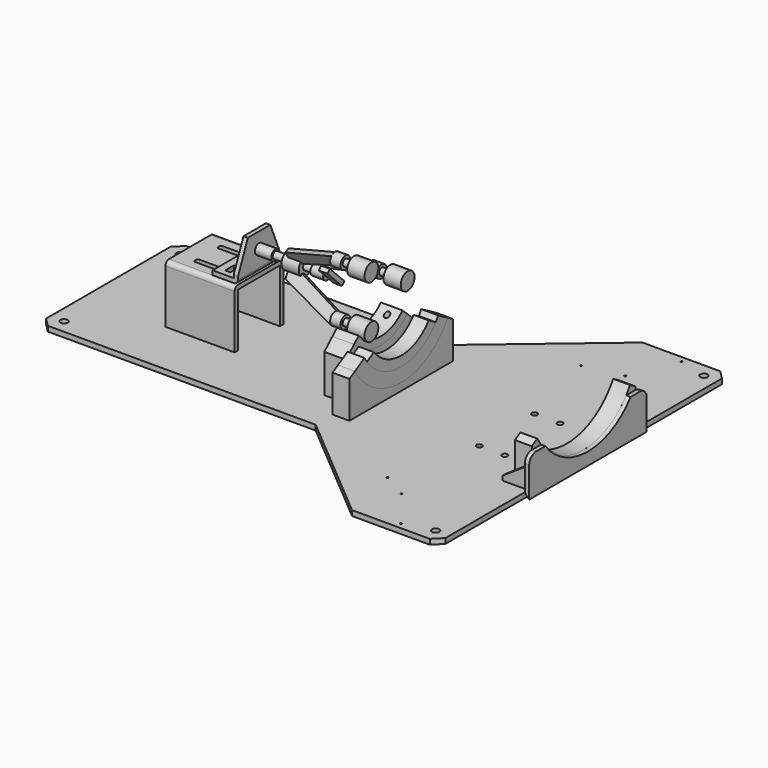
from build123d import *

# Parameters (mm, degrees)
F0_R      = 1
F0_R_2    = 3.2
F1_DEPTH  = 6
F3_W      = 29.5
F3_H      = 60.5
F3_W_2    = 6
F3_H_2    = 13
F4_DEPTH  = 5
F6_DEPTH  = 5
F7_R      = 5
F8_R      = 6
F8_R_2    = 4
F9_DEPTH  = 19
F10_R     = 4
F11_DEPTH = 15
F12_DEPTH = 15
F13_R     = 10
F13_R_2   = 4
F14_DEPTH = 20
F15_R     = 4
F16_DEPTH = 15
F17_DEPTH = 15
F18_R     = 4
F19_DEPTH = 10
F20_DEPTH = 20
F22_R     = 6
F23_DEPTH = 15
F25_DEPTH = 10
F26_ANGLE = 45
F28_R     = 10
F29_DEPTH = 20
F30_R     = 4
F31_DEPTH = 20
F33_R     = 7.2
F33_R_2   = 4
F34_DEPTH = 12
F35_W     = 15
F35_H     = 2.6824583655
F36_DEPTH = 5
F37_ANGLE = 120
F38_ANGLE = -120
F40_DEPTH = 19.5
F41_W     = 6
F41_H     = 3.5
F41_W_2   = 5
F41_H_2   = 60.5
F42_DEPTH = 5
F43_W     = 80
F43_H     = 62
F44_DEPTH = 5
F45_R     = 4.99999
F46_W     = 80
F46_H     = 62
F47_DEPTH = 5
F48_R     = 4.99999
F50_DEPTH = 5
F51_SIZE  = 4.99999
F53_DEPTH = 5
F57_DEPTH = 19.5
F58_DEPTH = 17.5
F61_DEPTH = 25
F62_DEPTH = 25
F63_DEPTH = 25
F64_R     = 3
F65_DEPTH = 137.3118891325
F64_R_2   = 4.25
F66_DEPTH = 25


# Not quite as in the source:
# - a fillet or chamfer is up to 0.001 mm smaller than in the source, because OpenCascade refuses the exact size


with BuildPart() as f1:
    # F0 (on Top) → F1 (new body)
    with BuildSketch(Plane.XY):
        Polygon((230, -200), (230, 200), (220, 210), (130, 210), (0, 100), (-310, 100), (-320, 90), (-320, -90), (-310, -100), (0, -100), (130, -210), (220, -210), align=None)
        with Locations((181, -203)):
            Circle(F0_R, mode=Mode.SUBTRACT)
        with Locations((115, -140)):
            Circle(F0_R, mode=Mode.SUBTRACT)
        with Locations((145, -157)):
            Circle(F0_R, mode=Mode.SUBTRACT)
        with Locations((8.75, -40)):
            Circle(F0_R_2, mode=Mode.SUBTRACT)
        with Locations((141.25, -40)):
            Circle(F0_R_2, mode=Mode.SUBTRACT)
        with Locations((170.75, -40)):
            Circle(F0_R_2, mode=Mode.SUBTRACT)
        with Locations((219.75, -40)):
            Circle(F0_R_2, mode=Mode.SUBTRACT)
        with Locations((8.75, 40)):
            Circle(F0_R_2, mode=Mode.SUBTRACT)
        with Locations((141.25, 40)):
            Circle(F0_R_2, mode=Mode.SUBTRACT)
        with Locations((170.75, 40)):
            Circle(F0_R_2, mode=Mode.SUBTRACT)
        with Locations((219.75, 40)):
            Circle(F0_R_2, mode=Mode.SUBTRACT)
        with Locations((115, 140)):
            Circle(F0_R, mode=Mode.SUBTRACT)
        with Locations((158.6559563875, 149.430975318)):
            Circle(F0_R, mode=Mode.SUBTRACT)
        with Locations((181, 203)):
            Circle(F0_R, mode=Mode.SUBTRACT)
    extrude(amount=F1_DEPTH)



with BuildPart() as f4:
    # F3 (on offset) → F4 (new body)
    with BuildSketch(Plane.XY.offset(73)):
        with Locations((-160.3453308344, 0)):
            Rectangle(F3_W, F3_H)
        with Locations((-163.0953308344, -16.8823601156)):
            Rectangle(F3_W_2, F3_H_2, mode=Mode.SUBTRACT)
        with Locations((-162.4798774719, 16.8823601156)):
            Rectangle(F3_W_2, F3_H_2, mode=Mode.SUBTRACT)
    extrude(amount=F4_DEPTH)

    # F5 (on face) → F6 (join)
    with BuildSketch(Plane.YZ.offset(-145.5953308344)):
        Polygon((-30.25, 78), (30.25, 78), (30.25, 81.6910490394), (16.2317510694, 115), (-16.2317510694, 115), (-30.25, 81.6910490394), align=None)
    extrude(amount=-F6_DEPTH)

    # F7
    f7_edges = [f4.edges().sort_by_distance(p)[0] for p in [
        (-145.595331, 0, 73),
    ]]
    fillet(f7_edges, radius=F7_R)

    # F41 (on face) → F42 (join)
    with BuildSketch(Plane(origin=(0, 0, 73), x_dir=(1, 0, 0), z_dir=(0, 0, -1))):
        with BuildLine():
            Line((-175.0953308344, 19.8823601156), (-175.0953308344, 30.25))
            Line((-175.0953308344, 30.25), (-225.5953308344, 30.25))
            Line((-225.5953308344, 30.25), (-225.5953308344, -30.25))
            Line((-225.5953308344, -30.25), (-175.0953308344, -30.25))
            Line((-175.0953308344, -30.25), (-175.0953308344, -19.8823601156))
            Line((-175.0953308344, -19.8823601156), (-203.5953308344, -19.8823601156))
            ThreePointArc((-203.5953308344, -19.8823601156), (-205.0095443968, -19.296573678), (-205.5953308344, -17.8823601156))
            Line((-205.5953308344, -17.8823601156), (-205.5953308344, -15.8823601156))
            ThreePointArc((-205.5953308344, -15.8823601156), (-205.0095443968, -14.4681465533), (-203.5953308344, -13.8823601156))
            Line((-203.5953308344, -13.8823601156), (-175.0953308344, -13.8823601156))
            Line((-175.0953308344, -13.8823601156), (-175.0953308344, 13.8823601156))
            Line((-175.0953308344, 13.8823601156), (-203.5953308344, 13.8823601156))
            ThreePointArc((-203.5953308344, 13.8823601156), (-205.0095443968, 14.4681465533), (-205.5953308344, 15.8823601156))
            Line((-205.5953308344, 15.8823601156), (-205.5953308344, 17.8823601156))
            ThreePointArc((-205.5953308344, 17.8823601156), (-205.0095443968, 19.296573678), (-203.5953308344, 19.8823601156))
            Line((-203.5953308344, 19.8823601156), (-175.0953308344, 19.8823601156))
        make_face()
        with BuildLine():
            Line((-150.5953308344, -30.25), (-150.5953308344, 30.25))
            Line((-150.5953308344, 30.25), (-175.0953308344, 30.25))
            Line((-175.0953308344, 30.25), (-175.0953308344, 19.8823601156))
            Line((-175.0953308344, 19.8823601156), (-166.0953308344, 19.8823601156))
            Line((-166.0953308344, 19.8823601156), (-166.0953308344, 23.3823601156))
            Line((-166.0953308344, 23.3823601156), (-160.0953308344, 23.3823601156))
            Line((-160.0953308344, 23.3823601156), (-160.0953308344, 19.8823601156))
            Line((-160.0953308344, 19.8823601156), (-157.5953308344, 19.8823601156))
            ThreePointArc((-157.5953308344, 19.8823601156), (-156.181117272, 19.296573678), (-155.5953308344, 17.8823601156))
            Line((-155.5953308344, 17.8823601156), (-155.5953308344, 15.8823601156))
            ThreePointArc((-155.5953308344, 15.8823601156), (-156.181117272, 14.4681465533), (-157.5953308344, 13.8823601156))
            Line((-157.5953308344, 13.8823601156), (-160.0953308344, 13.8823601156))
            Line((-160.0953308344, 13.8823601156), (-160.0953308344, 10.3823601156))
            Line((-160.0953308344, 10.3823601156), (-166.0953308344, 10.3823601156))
            Line((-166.0953308344, 10.3823601156), (-166.0953308344, 13.8823601156))
            Line((-166.0953308344, 13.8823601156), (-175.0953308344, 13.8823601156))
            Line((-175.0953308344, 13.8823601156), (-175.0953308344, -13.8823601156))
            Line((-175.0953308344, -13.8823601156), (-165.4798774719, -13.8823601156))
            Line((-165.4798774719, -13.8823601156), (-165.4798774719, -10.3823601156))
            Line((-165.4798774719, -10.3823601156), (-159.4798774719, -10.3823601156))
            Line((-159.4798774719, -10.3823601156), (-159.4798774719, -13.8823601156))
            Line((-159.4798774719, -13.8823601156), (-157.5953308344, -13.8823601156))
            ThreePointArc((-157.5953308344, -13.8823601156), (-156.181117272, -14.4681465533), (-155.5953308344, -15.8823601156))
            Line((-155.5953308344, -15.8823601156), (-155.5953308344, -17.8823601156))
            ThreePointArc((-155.5953308344, -17.8823601156), (-156.181117272, -19.296573678), (-157.5953308344, -19.8823601156))
            Line((-157.5953308344, -19.8823601156), (-159.4798774719, -19.8823601156))
            Line((-159.4798774719, -19.8823601156), (-159.4798774719, -23.3823601156))
            Line((-159.4798774719, -23.3823601156), (-165.4798774719, -23.3823601156))
            Line((-165.4798774719, -23.3823601156), (-165.4798774719, -19.8823601156))
            Line((-165.4798774719, -19.8823601156), (-175.0953308344, -19.8823601156))
            Line((-175.0953308344, -19.8823601156), (-175.0953308344, -30.25))
            Line((-175.0953308344, -30.25), (-150.5953308344, -30.25))
        make_face()
        with Locations((-162.4798774719, -21.6323601156)):
            Rectangle(F41_W, F41_H)
        with Locations((-162.4798774719, -12.1323601156)):
            Rectangle(F41_W, F41_H)
        with Locations((-163.0953308344, 12.1323601156)):
            Rectangle(F41_W, F41_H)
        with Locations((-163.0953308344, 21.6323601156)):
            Rectangle(F41_W, F41_H)
        with Locations((-148.0953308344, 0)):
            Rectangle(F41_W_2, F41_H_2)
    extrude(amount=F42_DEPTH)


with BuildPart() as f9:
    # F8 (on face) → F9 (new body)
    with BuildSketch(Plane.YZ.offset(-145.5953308344)):
        with Locations((0, 97)):
            Circle(F8_R)
        with Locations((0, 97)):
            Circle(F8_R_2, mode=Mode.SUBTRACT)
    extrude(amount=F9_DEPTH)


with BuildPart() as f11:
    # F10 (on face) → F11 (new body)
    with BuildSketch(Plane.YZ.offset(-126.5953308344)):
        with Locations((0, 97)):
            Circle(F10_R)
    extrude(amount=-F11_DEPTH)

    # F12 (add): a face of the model
    f12_faces = [f11.faces().sort_by_distance(p)[0] for p in [
        (-126.5953308344, 0, 97),
    ]]
    extrude(f12_faces, amount=F12_DEPTH)

    # F13 (on face) → F14 (join)
    with BuildSketch(Plane.YZ.offset(-111.5953308344)):
        with Locations((0, 97)):
            Circle(F13_R)
        with Locations((0, 97)):
            Circle(F13_R_2, mode=Mode.SUBTRACT)
        with Locations((0, 97)):
            Circle(F13_R_2)
    extrude(amount=F14_DEPTH)

    # F15 (on face) → F16 (cut)
    with BuildSketch(Plane.YZ.offset(-91.5953308344)):
        with Locations((0, 97)):
            Circle(F15_R)
    extrude(amount=-F16_DEPTH, mode=Mode.SUBTRACT)

    # F15 (on face) → F17 (cut)
    with BuildSketch(Plane.YZ.offset(-91.5953308344)):
        with BuildLine():
            ThreePointArc((-2.6761656733, 106.6352549156), (-5, 105.6602540378), (-7.0062926922, 104.1352549156))
            Line((-7.0062926922, 104.1352549156), (-5.6650635095, 101.8121778265))
            Line((-5.6650635095, 101.8121778265), (-1.3349364905, 104.3121778265))
            Line((-1.3349364905, 104.3121778265), (-2.6761656733, 106.6352549156))
        make_face()
        with BuildLine():
            ThreePointArc((-7.0062926922, 89.8647450844), (-5, 88.3397459622), (-2.6761656733, 87.3647450844))
            Line((-2.6761656733, 87.3647450844), (-1.3349364905, 89.6878221735))
            Line((-1.3349364905, 89.6878221735), (-5.6650635095, 92.1878221735))
            Line((-5.6650635095, 92.1878221735), (-7.0062926922, 89.8647450844))
        make_face()
        with BuildLine():
            Line((7, 94.5), (9.6824583655, 94.5))
            ThreePointArc((9.6824583655, 94.5), (9.9202969627, 95.7399570752), (10, 97))
            ThreePointArc((10, 97), (9.9202969627, 98.2600429248), (9.6824583655, 99.5))
            Line((9.6824583655, 99.5), (7, 99.5))
            Line((7, 99.5), (7, 94.5))
        make_face()
    extrude(amount=-F17_DEPTH, mode=Mode.SUBTRACT)


with BuildPart() as f19:
    # F18 (on face) → F19 (new body)
    with BuildSketch(Plane.YZ.offset(-91.5953308344)):
        with Locations((0, 97)):
            Circle(F18_R)
    extrude(amount=-F19_DEPTH)

    # F20 (add): a face of the model
    f20_faces = [f19.faces().sort_by_distance(p)[0] for p in [
        (-91.5953308344, 0, 97),
    ]]
    extrude(f20_faces, amount=F20_DEPTH)


with BuildPart() as f23:
    # F22 (on offset) → F23 (new body)
    with BuildSketch(Plane.YZ.offset(-81.5953308344)):
        with Locations((0, 97)):
            Circle(F22_R)
    extrude(amount=F23_DEPTH)

    # F24 (on face) → F25 (join)
    with BuildSketch(Plane.YZ.offset(-66.5953308344)):
        with BuildLine():
            Line((2.5, 112), (-2.5, 112))
            Line((-2.5, 112), (-2.5, 102.4543560573))
            ThreePointArc((-2.5, 102.4543560573), (0, 103), (2.5, 102.4543560573))
            Line((2.5, 102.4543560573), (2.5, 112))
        make_face()
        with BuildLine():
            ThreePointArc((2.5, 102.4543560573), (0, 103), (-2.5, 102.4543560573))
            Line((-2.5, 102.4543560573), (-2.5, 91.5456439427))
            ThreePointArc((-2.5, 91.5456439427), (0, 91), (2.5, 91.5456439427))
            Line((2.5, 91.5456439427), (2.5, 102.4543560573))
        make_face()
        with BuildLine():
            ThreePointArc((2.5, 91.5456439427), (0, 91), (-2.5, 91.5456439427))
            Line((-2.5, 91.5456439427), (-2.5, 82))
            Line((-2.5, 82), (2.5, 82))
            Line((2.5, 82), (2.5, 91.5456439427))
        make_face()
    extrude(amount=F25_DEPTH)


with BuildPart() as f23_1:
    # F26: moved
    add(f23.part.rotate(Axis((-91.5953308344, 0, 97), (1, 0, 0)), F26_ANGLE))


with BuildPart() as f29:
    # F28 (on offset) → F29 (new body)
    with BuildSketch(Plane.YZ.offset(-1.5953308344)):
        with Locations((-17.5, 127.3108891325)):
            Circle(F28_R)
    extrude(amount=-F29_DEPTH)


with BuildPart() as f29b:
    # F28 (on offset) → F29, piece 2 (new body)
    with BuildSketch(Plane.YZ.offset(-1.5953308344)):
        with Locations((35, 97)):
            Circle(F28_R)
    extrude(amount=-F29_DEPTH)


with BuildPart() as f29c:
    # F28 (on offset) → F29, piece 3 (new body)
    with BuildSketch(Plane.YZ.offset(-1.5953308344)):
        with Locations((-17.5, 66.6891108675)):
            Circle(F28_R)
    extrude(amount=-F29_DEPTH)


with BuildPart() as f31:
    # F30 (on face) → F31 (new body)
    with BuildSketch(Plane(origin=(-21.5953308344, 0, 0), x_dir=(0, -1, 0), z_dir=(-1, 0, 0))):
        with Locations((17.5, 66.6891108675)):
            Circle(F30_R)
    extrude(amount=F31_DEPTH)


with BuildPart() as f31b:
    # F30 (on face) → F31, piece 2 (new body)
    with BuildSketch(Plane(origin=(-21.5953308344, 0, 0), x_dir=(0, -1, 0), z_dir=(-1, 0, 0))):
        with Locations((-35, 97)):
            Circle(F30_R)
    extrude(amount=F31_DEPTH)


with BuildPart() as f31c:
    # F30 (on face) → F31, piece 3 (new body)
    with BuildSketch(Plane(origin=(-21.5953308344, 0, 0), x_dir=(0, -1, 0), z_dir=(-1, 0, 0))):
        with Locations((17.5, 127.3108891325)):
            Circle(F30_R)
    extrude(amount=F31_DEPTH)


with BuildPart() as f34:
    # F33 (on offset) → F34 (new body)
    with BuildSketch(Plane(origin=(-31.5953308344, 0, 0), x_dir=(0, -1, 0), z_dir=(-1, 0, 0))):
        with Locations((17.5, 127.3108891325)):
            Circle(F33_R)
        with Locations((17.5, 127.3108891325)):
            Circle(F33_R_2, mode=Mode.SUBTRACT)
    extrude(amount=F34_DEPTH)


with BuildPart() as f34b:
    # F33 (on offset) → F34, piece 2 (new body)
    with BuildSketch(Plane(origin=(-31.5953308344, 0, 0), x_dir=(0, -1, 0), z_dir=(-1, 0, 0))):
        with Locations((17.5, 66.6891108675)):
            Circle(F33_R)
        with Locations((17.5, 66.6891108675)):
            Circle(F33_R_2, mode=Mode.SUBTRACT)
    extrude(amount=F34_DEPTH)


with BuildPart() as f34c:
    # F33 (on offset) → F34, piece 3 (new body)
    with BuildSketch(Plane(origin=(-31.5953308344, 0, 0), x_dir=(0, -1, 0), z_dir=(-1, 0, 0))):
        with Locations((-35, 97)):
            Circle(F33_R)
        with Locations((-35, 97)):
            Circle(F33_R_2, mode=Mode.SUBTRACT)
    extrude(amount=F34_DEPTH)


with BuildPart() as f36:
    # F35 (on face) → F36 (new body)
    with BuildSketch(Plane(origin=(0, 39.8371685741, 23), x_dir=(-1, 0, 0), z_dir=(0, 0.8660254038, 0.5))):
        Polygon((43.5953308344, 111.8044641671), (91.5953308344, 91.0044641671), (91.5953308344, 93.6869225326), (106.5953308344, 93.6869225326), (106.5953308344, 101.0044641671), (43.5953308344, 126.2044641671), align=None)
        with Locations((99.0953308344, 92.3456933498)):
            Rectangle(F35_W, F35_H)
    extrude(amount=F36_DEPTH)


with BuildPart() as f37_1:
    # F37: copy of F36
    add(f36.part.rotate(Axis((-111.5953308344, 0, 97), (-1, 0, 0)), F37_ANGLE))


with BuildPart() as f38_1:
    # F38: copy of F36
    add(f36.part.rotate(Axis((-111.5953308344, 0, 97), (-1, 0, 0)), F38_ANGLE))


with BuildPart() as f40:
    # F39 (on face) → F40 (new body)
    with BuildSketch(Plane.YZ.offset(230)):
        with BuildLine():
            Line((-75, 48.6987298108), (-75, 6))
            Line((-75, 6), (75, 6))
            Line((75, 6), (75, 48.6987298108))
            Line((75, 48.6987298108), (67.1169687933, 53.25))
            ThreePointArc((67.1169687933, 53.25), (0, 14.5), (-67.1169687933, 53.25))
            Line((-67.1169687933, 53.25), (-75, 48.6987298108))
        make_face()
    extrude(amount=-F40_DEPTH)


with BuildPart() as f1_1:
    add(f1.part)

    add(f4.part)  # F44 merges F4
    # F43 (on face) → F44 (join)
    with BuildSketch(Plane.XZ.offset(30.25)):
        with Locations((-185.5953308344, 37)):
            Rectangle(F43_W, F43_H)
        Polygon((-145.5953308344, 68), (-145.5953308344, 73), (-150.5953308344, 73), (-175.0953308344, 73), (-225.5953308344, 73), (-225.5953308344, 68), align=None)
    extrude(amount=F44_DEPTH)

    # F45 (radius 5 in the source; OpenCascade refuses exactly that, so slightly less here)
    f45_edges = [f1_1.edges().sort_by_distance(p)[0] for p in [
        (-185.595331, -35.25, 73),
    ]]
    fillet(f45_edges, radius=F45_R)

    # F46 (on face) → F47 (join)
    with BuildSketch(Plane(origin=(0, 30.25, 0), x_dir=(-1, 0, 0), z_dir=(0, 1, 0))):
        with Locations((185.5953308344, 37)):
            Rectangle(F46_W, F46_H)
        Polygon((225.5953308344, 68), (225.5953308344, 73), (175.0953308344, 73), (150.5953308344, 73), (145.5953308344, 73), (145.5953308344, 68), align=None)
    extrude(amount=F47_DEPTH)

    # F48 (radius 5 in the source; OpenCascade refuses exactly that, so slightly less here)
    f48_edges = [f1_1.edges().sort_by_distance(p)[0] for p in [
        (-185.595331, 35.25, 73),
    ]]
    fillet(f48_edges, radius=F48_R)


with BuildPart() as f50:
    # F49 (on face) → F50 (new body)
    with BuildSketch(Plane.YZ.offset(230)):
        with BuildLine():
            Line((-85, 0), (85, 0))
            Line((85, 0), (85, 35))
            ThreePointArc((85, 35), (82.0710678119, 42.0710678119), (75, 45))
            Line((75, 45), (75, 6))
            Line((75, 6), (-75, 6))
            Line((-75, 6), (-75, 45))
            ThreePointArc((-75, 45), (-82.0710678119, 42.0710678119), (-85, 35))
            Line((-85, 35), (-85, 0))
        make_face()
        with BuildLine():
            Line((75, 6), (75, 45))
            Line((75, 45), (61.6218305473, 45))
            ThreePointArc((61.6218305473, 45), (0, 14.5), (-61.6218305473, 45))
            Line((-61.6218305473, 45), (-75, 45))
            Line((-75, 45), (-75, 6))
            Line((-75, 6), (75, 6))
        make_face()
    extrude(amount=F50_DEPTH)

    # F51 (size 5 in the source; OpenCascade refuses exactly that, so slightly less here)
    f51_edges = [f50.edges().sort_by_distance(p)[0] for p in [
        (230, 0, 0),
    ]]
    chamfer(f51_edges, length=F51_SIZE)


with BuildPart() as f53:
    # F52 (on face) → F53 (new body)
    with BuildSketch(Plane.XZ.offset(75)):
        Polygon((200, 6), (210.5, 6), (210.5, 18), (200, 11), align=None)
        Polygon((210.5, 6), (230, 6), (230, 31), (210.5, 18), align=None)
    extrude(amount=F53_DEPTH)


with BuildPart() as f54_1:
    # F54: copy of F53
    add(f53.part.moved(Location((0, 155, 0))))


with BuildPart() as f55_1:
    # F55: copy of F40
    add(f40.part.moved(Location((-211, 0, 0))))


with BuildPart() as f57:
    # F56 (on face) → F57 (new body)
    with BuildSketch(Plane.YZ.offset(19)):
        with BuildLine():
            Line((-53.2605623327, 61.25), (-67.1169687933, 53.25))
            ThreePointArc((-67.1169687933, 53.25), (0, 14.5), (67.1169687933, 53.25))
            Line((67.1169687933, 53.25), (53.2605623327, 61.25))
            ThreePointArc((53.2605623327, 61.25), (51.5597557341, 58.4762533621), (49.7146348004, 55.7963387671))
            ThreePointArc((49.7146348004, 55.7963387671), (0, 30.5), (-49.7146348004, 55.7963387671))
            ThreePointArc((-49.7146348004, 55.7963387671), (-51.5597557341, 58.4762533621), (-53.2605623327, 61.25))
        make_face()
    extrude(amount=-F57_DEPTH)


with BuildPart() as f58:
    # F56 (on face) → F58 (new body)
    with BuildSketch(Plane.YZ.offset(19)):
        with BuildLine():
            Line((-39.6862859915, 61.5862086514), (-49.7146348004, 55.7963387671))
            ThreePointArc((-49.7146348004, 55.7963387671), (0, 30.5), (49.7146348004, 55.7963387671))
            Line((49.7146348004, 55.7963387671), (39.6862859915, 61.5862086514))
            ThreePointArc((39.6862859915, 61.5862086514), (0, 42), (-39.6862859915, 61.5862086514))
        make_face()
    extrude(amount=-F58_DEPTH)


with BuildPart() as f61:
    # F60 (on offset) → F61 (new body)
    with BuildSketch(Plane.YZ.offset(-30)):
        with BuildLine():
            Line((-50, 6), (50, 6))
            Line((50, 6), (50, 50.1785305656))
            ThreePointArc((50, 50.1785305656), (0, 28.5), (-50, 50.1785305656))
            Line((-50, 50.1785305656), (-50, 6))
        make_face()
    extrude(amount=F61_DEPTH)


with BuildPart() as f62:
    # F60 (on offset) → F62 (new body)
    with BuildSketch(Plane.YZ.offset(-30)):
        with BuildLine():
            ThreePointArc((-50, 50.1785305656), (0, 28.5), (50, 50.1785305656))
            Line((50, 50.1785305656), (38.3211678832, 61.1149321853))
            ThreePointArc((38.3211678832, 61.1149321853), (0, 44.5), (-38.3211678832, 61.1149321853))
            Line((-38.3211678832, 61.1149321853), (-50, 50.1785305656))
        make_face()
    extrude(amount=F62_DEPTH)


with BuildPart() as f63:
    # F60 (on offset) → F63 (new body)
    with BuildSketch(Plane.YZ.offset(-30)):
        with BuildLine():
            ThreePointArc((-38.3211678832, 61.1149321853), (0, 44.5), (38.3211678832, 61.1149321853))
            Line((38.3211678832, 61.1149321853), (31.7518248175, 67.2666580964))
            ThreePointArc((31.7518248175, 67.2666580964), (0, 53.5), (-31.7518248175, 67.2666580964))
            Line((-31.7518248175, 67.2666580964), (-38.3211678832, 61.1149321853))
        make_face()
    extrude(amount=F63_DEPTH)


with BuildPart() as f65_tool:
    # F64 (on face) → F65 (new body, through all)
    with BuildSketch(Plane(origin=(0, 0, 0), x_dir=(1, 0, 0), z_dir=(0, 0, -1))):
        with Locations((-17.5, 25)):
            Circle(F64_R)
        with Locations((-17.5, -25)):
            Circle(F64_R)
    extrude(amount=-F65_DEPTH)


with BuildPart() as f1_2:
    add(f1_1.part)

    # F65: cut by f65_tool
    add(f65_tool.part, mode=Mode.SUBTRACT)

    # F64 (on face) → F66 (cut)
    with BuildSketch(Plane(origin=(0, 0, 0), x_dir=(1, 0, 0), z_dir=(0, 0, -1))):
        with Locations((-304, 84)):
            Circle(F64_R_2)
        with Locations((-304, -84)):
            Circle(F64_R_2)
        with Locations((214, -194)):
            Circle(F64_R_2)
        with Locations((214, 194)):
            Circle(F64_R_2)
    extrude(amount=-F66_DEPTH, mode=Mode.SUBTRACT)


with BuildPart() as f61_1:
    add(f61.part)

    # F65: cut by f65_tool
    add(f65_tool.part, mode=Mode.SUBTRACT)


with BuildPart() as f62_1:
    add(f62.part)

    # F65: cut by f65_tool
    add(f65_tool.part, mode=Mode.SUBTRACT)


with BuildPart() as f63_1:
    add(f63.part)

    # F65: cut by f65_tool
    add(f65_tool.part, mode=Mode.SUBTRACT)


solid = Compound([f9.part, f11.part, f19.part, f23_1.part, f29.part, f29b.part, f29c.part, f31.part, f31b.part, f31c.part, f34.part, f34b.part, f34c.part, f36.part, f37_1.part, f38_1.part, f40.part, f50.part, f53.part, f54_1.part, f55_1.part, f57.part, f58.part, f1_2.part, f61_1.part, f62_1.part, f63_1.part])
